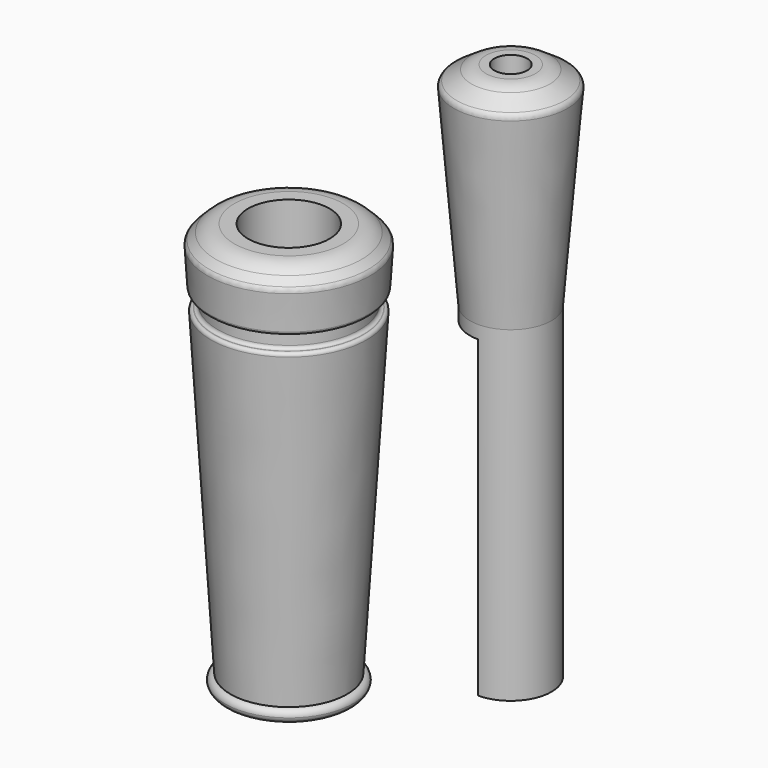
from build123d import *

# Parameters (mm, degrees)
F2_R     = 7.9375
F3_DEPTH = 79.376
F7_DEPTH = 60.96
F8_R     = 3.175
F9_DEPTH = 95.25
F10_R    = 5.08
F11_R    = 1.27
F12_R    = 5.08
F13_R    = 1.27
F14_R    = 0.635
F15_R    = 0.635
F18_R    = 0.508


# Not quite as in the source:
# - a fillet or chamfer that OpenCascade refuses, or shapes differently, is made with other operations: its cross-section is extruded or revolved along the edge and cut away or added


with BuildPart() as f1:
    # F0 (on Front) → F1 (revolve)
    with BuildSketch(Plane.XZ):
        Polygon((-41.9936563492, 0), (-45.1686563492, -3.175), (-29.2936563492, -3.175), (-29.2936563492, 0), align=None)
        Polygon((-29.2936563492, -3.175), (-45.1686563492, -3.175), (-44.6791771825, -11.1125), (-43.0916771825, -11.1125), (-43.0916771825, -12.7), (-29.2936563492, -12.7), align=None)
        Polygon((-29.2936563492, -76.835), (-29.2936563492, -12.7), (-43.0916771825, -12.7), (-43.0916771825, -14.2875), (-44.4833855158, -14.2875), (-40.6262896825, -76.835), align=None)
        Polygon((-29.2936563492, -79.375), (-29.2936563492, -76.835), (-40.6262896825, -76.835), (-40.4696563492, -79.375), align=None)
        Polygon((-40.4696563492, -79.375), (-40.6262896825, -76.835), (-41.7396563492, -76.835), (-41.7396563492, -79.375), align=None)
    revolve(axis=Axis((-29.2936563492, 0, -41.275), (0, 0, -1)))

    # F2 (on face) → F3 (cut, through all)
    with BuildSketch(Plane.XY):
        with Locations((-29.2936563492, 0)):
            Circle(F2_R)
    extrude(amount=-F3_DEPTH, mode=Mode.SUBTRACT)

    # F12
    f12_edges = [f1.edges().sort_by_distance(p)[0] for p in [
        (-16.593656, 0, 0),
    ]]
    fillet(f12_edges, radius=F12_R)

    # F13
    f13_edges = [f1.edges().sort_by_distance(p)[0] for p in [
        (-13.418656, 0, -3.175),
    ]]
    fillet(f13_edges, radius=F13_R)

    # F14
    f14_edges = [f1.edges().sort_by_distance(p)[0] for p in [
        (-14.103927, 0, -14.2875),
        (-13.908136, 0, -11.1125),
    ]]
    fillet(f14_edges, radius=F14_R)

    # F15
    f15_edges = [f1.edges().sort_by_distance(p)[0] for p in [
        (-15.495636, 0, -14.2875),
        (-14.505183, 0, -11.1125),
    ]]
    fillet(f15_edges, radius=F15_R)

    # F16: fillet of radius 1.27 on 1 edges, made by hand

    # F16_s1 → F16_t2 (revolve, cut)
    with BuildSketch(Plane.XZ):
        with BuildLine():
            ThreePointArc((-40.6262896825, -76.835), (-41.4214505321, -77.2544782457), (-41.7396563492, -78.0953039312))
            Line((-41.7396563492, -78.0953039312), (-41.7650563492, -78.0953039312))
            Line((-41.7650563492, -78.0953039312), (-41.7650563492, -76.835))
            Line((-41.7650563492, -76.835), (-41.7396563492, -76.8096))
            ThreePointArc((-41.7396563492, -76.8096), (-41.1829730158, -76.8096), (-40.6294223492, -76.8097939214))
            Line((-40.6294223492, -76.8097939214), (-40.6262896825, -76.835))
        make_face()
    revolve(axis=Axis((-29.2936563492, 0, -76.835), (0, 0, -1)), mode=Mode.SUBTRACT)

    # F17: fillet of radius 1.524 on 1 edges, made by hand

    # F17_s1 → F17_t2 (revolve, cut)
    with BuildSketch(Plane.XZ):
        with BuildLine():
            ThreePointArc((-41.7396563492, -78.0953039312), (-41.2228511914, -79.0117961042), (-40.2353652905, -79.375))
            Line((-40.2353652905, -79.375), (-40.2353652905, -79.40548))
            Line((-40.2353652905, -79.40548), (-41.7396563492, -79.40548))
            Line((-41.7396563492, -79.40548), (-41.7701363492, -79.375))
            ThreePointArc((-41.7701363492, -79.375), (-41.7701363492, -78.7351519656), (-41.7697421704, -78.1001900098))
            Line((-41.7697421704, -78.1001900098), (-41.7396563492, -78.0953039312))
        make_face()
    revolve(axis=Axis((-29.2936563492, 0, -79.375), (0, 0, -1)), mode=Mode.SUBTRACT)

    # F18
    f18_edges = [f1.edges().sort_by_distance(p)[0] for p in [
        (-37.231156, 0, -79.375),
    ]]
    fillet(f18_edges, radius=F18_R)


with BuildPart() as f5:
    # F4 (on Front) → F5 (revolve)
    with BuildSketch(Plane.XZ):
        Polygon((13.8481526896, -63.5), (13.8481526896, 0), (13.8481526896, 38.1), (2.7356526896, 38.1), (5.9106526896, 0), (5.9106526896, -63.5), align=None)
        Polygon((2.7356526896, 38.1), (13.8481526896, 38.1), (13.8481526896, 41.275), (7.4981526896, 41.275), align=None)
    revolve(axis=Axis((13.8481526896, 0, 19.05), (0, 0, 1)))

    # F6 (on face) → F7 (cut)
    with BuildSketch(Plane(origin=(0, 0, -63.5), x_dir=(1, 0, 0), z_dir=(0, 0, -1))):
        with BuildLine():
            Line((13.8481526896, -7.9375), (13.8481526896, 7.9375))
            ThreePointArc((13.8481526896, 7.9375), (5.9106526896, 0), (13.8481526896, -7.9375))
        make_face()
    extrude(amount=-F7_DEPTH, mode=Mode.SUBTRACT)

    # F8 (on face) → F9 (cut)
    with BuildSketch(Plane.XY.offset(41.275)):
        with Locations((13.8481526896, 0)):
            Circle(F8_R)
    extrude(amount=-F9_DEPTH, mode=Mode.SUBTRACT)

    # F10
    f10_edges = [f5.edges().sort_by_distance(p)[0] for p in [
        (20.198153, 0, 41.275),
    ]]
    fillet(f10_edges, radius=F10_R)

    # F11
    f11_edges = [f5.edges().sort_by_distance(p)[0] for p in [
        (24.960653, 0, 38.1),
    ]]
    fillet(f11_edges, radius=F11_R)


solid = Compound([f1.part, f5.part])
